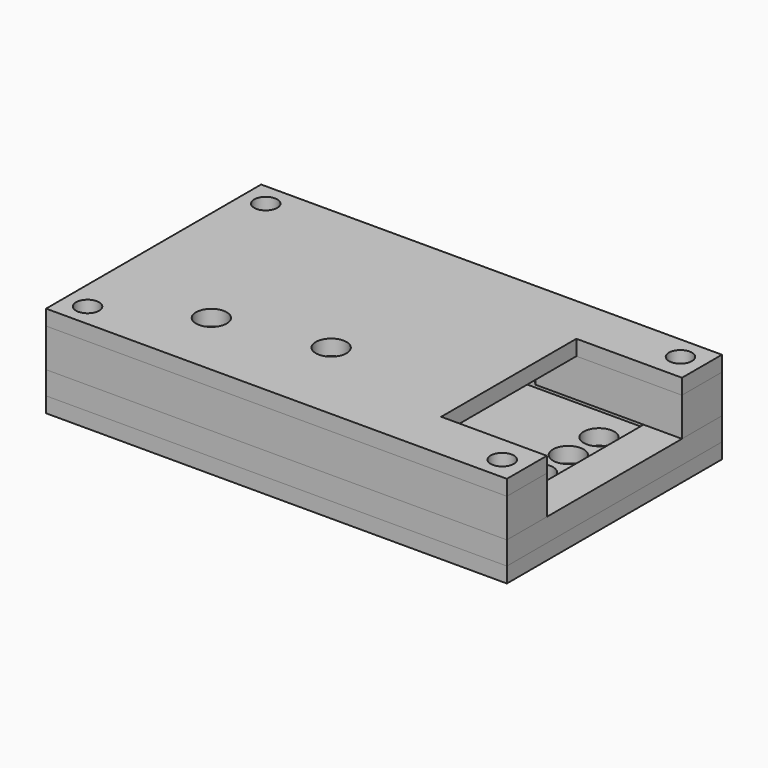
from build123d import *

# Parameters (mm, degrees)
F0_W      = 60
F0_H      = 35.000001
F0_R      = 1.5
F1_DEPTH  = 2
F3_R      = 1.5
F4_DEPTH  = 3
F5_R      = 2.000001
F6_DEPTH  = 2
F8_R      = 1.5
F9_DEPTH  = 5
F11_R     = 1.5
F11_R_2   = 2.000001
F12_DEPTH = 2


with BuildPart() as f1:
    # F0 (on Top) → F1 (new body)
    with BuildSketch(Plane.XY):
        with Locations((0, -5e-07)):
            Rectangle(F0_W, F0_H)
        with Locations((-27.000001, -14.500002)):
            Circle(F0_R, mode=Mode.SUBTRACT)
        with Locations((27, -14.500002)):
            Circle(F0_R, mode=Mode.SUBTRACT)
        with Locations((-27.000001, 14.499999)):
            Circle(F0_R, mode=Mode.SUBTRACT)
        with Locations((27, 14.499999)):
            Circle(F0_R, mode=Mode.SUBTRACT)
    extrude(amount=F1_DEPTH)


with BuildPart() as f4:
    # F3 (on offset) → F4 (new body)
    with BuildSketch(Plane.XY.offset(2)):
        Polygon((24.000001, -11.899999), (24.000001, -12.000002), (-23.999999, -12.000002), (-23.999999, -11.700002), (-24.7, -11.000001), (-25, -11.000001), (-25, -6.5), (-30, -6.5), (-30, -17.500001), (30, -17.500001), (30, 11.000001), (30, 17.5), (-30, 17.5), (-30, 6.499999), (-25, 6.499999), (-25, 10.999998), (-24.6, 10.999998), (-23.999999, 11.599999), (-23.999999, 11.999999), (24.000001, 11.999999), (24.000001, 11.899999), (24.400001, 11.5), (24.999999, 11.5), (24.999999, -11.5), (24.400001, -11.5), align=None)
        with Locations((-27.000001, -14.500002)):
            Circle(F3_R, mode=Mode.SUBTRACT)
        with Locations((27, -14.500002)):
            Circle(F3_R, mode=Mode.SUBTRACT)
        with Locations((-27.000001, 14.499999)):
            Circle(F3_R, mode=Mode.SUBTRACT)
        with Locations((27, 14.499999)):
            Circle(F3_R, mode=Mode.SUBTRACT)
    extrude(amount=F4_DEPTH)


with BuildPart() as f6:
    # F5 (on offset) → F6 (new body)
    with BuildSketch(Plane.XY.offset(2)):
        Polygon((-23.999999, -10.999999), (-23.999999, -12), (24.000001, -12), (24.000001, -11.499998), (24.999999, -11.499998), (24.999999, 11.500002), (24.000001, 11.500002), (24.000001, 12.000001), (-23.999999, 12.000001), (-23.999999, 11), (-25, 11), (-25, -10.999999), align=None)
        with Locations((22, -7.499999)):
            Circle(F5_R, mode=Mode.SUBTRACT)
        with Locations((22, -2.499755)):
            Circle(F5_R, mode=Mode.SUBTRACT)
        with Locations((22, 2.500002)):
            Circle(F5_R, mode=Mode.SUBTRACT)
        with Locations((22, 7.500246)):
            Circle(F5_R, mode=Mode.SUBTRACT)
    extrude(amount=F6_DEPTH)


with BuildPart() as f9:
    # F8 (on offset) → F9 (new body)
    with BuildSketch(Plane.XY.offset(5)):
        Polygon((-22.999999, 10.499999), (-22.999999, 11.799999), (-19.049999, 11.799999), (-19.049999, 9.449999), (-15.125, 9.449999), (-15.125, 5.899998), (-8.5, 5.899998), (-8.5, -1.5), (-8.5, -3.775002), (-9.999999, -3.775002), (-9.999999, -4.900001), (-9.999999, -12.000002), (-22.000001, -12.000002), (-22.000001, -10.5), (-23.300001, -10.5), (-23.300001, -6.5), (-30, -6.5), (-30, -17.500001), (30, -17.500001), (30, -11.000001), (18.000001, -11.000001), (18.000001, -11.5), (15.500001, -11.5), (10.000001, -11.5), (2.750001, -11.5), (1.65, -11.5), (1.65, -12.000002), (1.399998, -12.000002), (-5.500001, -12.000002), (-5.500001, -0.950001), (-5.500001, -0.275001), (1.500001, -0.275001), (1.500001, 1.399999), (3.225001, 1.399999), (3.225001, -0.425001), (5.424999, -0.425001), (5.424999, 1.199997), (5.65, 1.199997), (9.274999, 1.199997), (9.274999, 2.974998), (9.249998, 2.999999), (7.824999, 2.999999), (7.824999, 6.374998), (9.4, 6.374998), (9.4, 7.649997), (8.750001, 8.299996), (8.750001, 11.5), (10.424999, 11.5), (10.924998, 11.000001), (17.2, 11.000001), (30, 11.000001), (30, 17.5), (-30, 17.5), (-30, 6.499999), (-26, 6.499999), (-24.6, 6.499999), (-24.6, 10.499999), align=None)
        with Locations((-27.000001, -14.500002)):
            Circle(F8_R, mode=Mode.SUBTRACT)
        with Locations((27, -14.500002)):
            Circle(F8_R, mode=Mode.SUBTRACT)
        Polygon((0.025, 5.349997), (0.025, 1.849996), (-6.324998, 1.849996), (-6.424997, 1.949996), (-6.424997, 5.199997), (-6.274998, 5.349997), align=None, mode=Mode.SUBTRACT)
        with Locations((-27.000001, 14.499999)):
            Circle(F8_R, mode=Mode.SUBTRACT)
        with Locations((27, 14.499999)):
            Circle(F8_R, mode=Mode.SUBTRACT)
    extrude(amount=F9_DEPTH)


with BuildPart() as f12:
    # F11 (on offset) → F12 (new body)
    with BuildSketch(Plane.XY.offset(10)):
        Polygon((-30, 17.5), (-30, -17.500001), (30, -17.500001), (30, -11.000001), (16.249999, -11.000001), (16.249999, 11.000001), (30, 11.000001), (30, 17.5), align=None)
        with Locations((-27.000001, -14.500002)):
            Circle(F11_R, mode=Mode.SUBTRACT)
        with Locations((-15.600001, -8.600001)):
            Circle(F11_R_2, mode=Mode.SUBTRACT)
        with Locations((-2, -6.100001)):
            Circle(F11_R_2, mode=Mode.SUBTRACT)
        with Locations((27, -14.500002)):
            Circle(F11_R, mode=Mode.SUBTRACT)
        with Locations((-27.000001, 14.499999)):
            Circle(F11_R, mode=Mode.SUBTRACT)
        with Locations((27, 14.499999)):
            Circle(F11_R, mode=Mode.SUBTRACT)
    extrude(amount=F12_DEPTH)


solid = Compound([f1.part, f4.part, f6.part, f9.part, f12.part])
